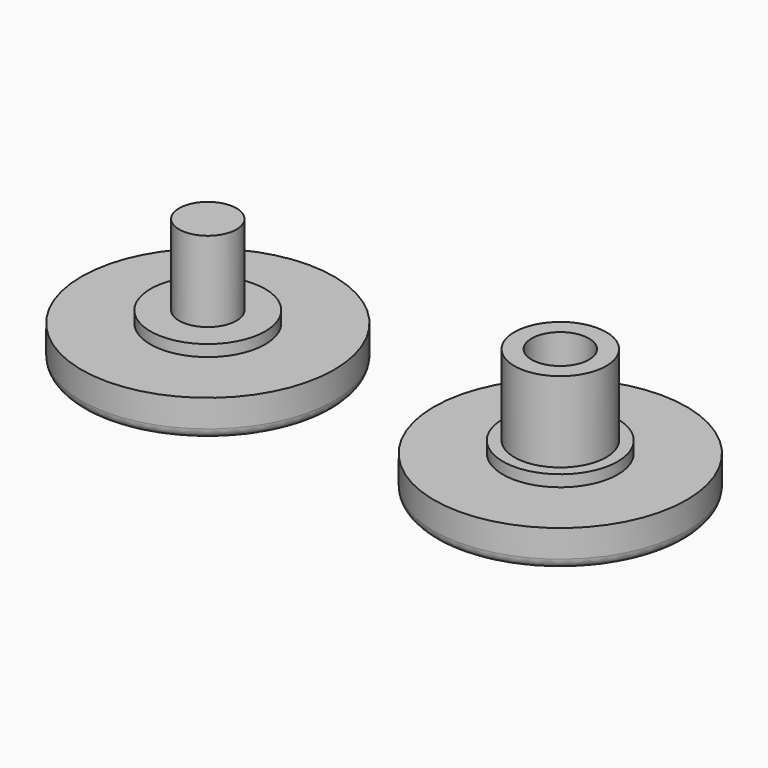
from build123d import *

# Parameters (mm, degrees)
F0_R      = 11
F1_DEPTH  = 3.5
F2_R      = 5
F3_DEPTH  = 1
F4_R      = 4
F5_DEPTH  = 7
F6_R      = 1.3518679975
F7_DEPTH  = 32.3
F11_R     = 0.9092071391
F13_R     = 2.5
F14_DEPTH = 7
F15_R     = 4
F15_R_2   = 2.5
F16_DEPTH = 7


# Not quite as in the source:
# - a fillet or chamfer that OpenCascade refuses, or shapes differently, is made with other operations: its cross-section is extruded or revolved along the edge and cut away or added
# - a feature names something its author has since deleted; it is built from what else it names


with BuildPart() as f1:
    # F0 (on Top) → F1 (new body)
    with BuildSketch(Plane.XY):
        with Locations((59.4149753451, 64.0600547194)):
            Circle(F0_R)
    extrude(amount=F1_DEPTH)

    # F2 (on face) → F3 (join)
    with BuildSketch(Plane.XY.offset(3.5)):
        with Locations((59.4149753451, 64.0600547194)):
            Circle(F2_R)
    extrude(amount=F3_DEPTH)

    # F4 (on face) → F5 (join)
    with BuildSketch(Plane.XY.offset(4.5)):
        with Locations((59.4149753451, 64.0600547194)):
            Circle(F4_R)
    extrude(amount=F5_DEPTH)

    # F6 (on face) → F7 (join)
    with BuildSketch(Plane(origin=(0, 0, 0), x_dir=(1, 0, 0), z_dir=(0, 0, -1))):
        with Locations((59.4149753451, -64.0600547194)):
            Circle(F6_R)
    extrude(amount=F7_DEPTH)

    # F8 (on face) → F9 (revolve, cut)
    with BuildSketch(Plane(origin=(0, 0, -32.3), x_dir=(1, 0, 0), z_dir=(0, 0, -1))):
        with BuildLine():
            Line((60.7668433426, -64.0600547194), (93.4149753451, -64.0600547194))
            ThreePointArc((93.4149753451, -64.0600547194), (59.4149753451, -30.0600547194), (25.4149753451, -64.0600547194))
            Line((25.4149753451, -64.0600547194), (58.0631073476, -64.0600547194))
            ThreePointArc((58.0631073476, -64.0600547194), (59.4149753451, -62.7081867219), (60.7668433426, -64.0600547194))
        make_face()
        with BuildLine():
            Line((59.4149753451, -64.0600547194), (60.7668433426, -64.0600547194))
            ThreePointArc((60.7668433426, -64.0600547194), (59.4149753451, -62.7081867219), (58.0631073476, -64.0600547194))
            Line((58.0631073476, -64.0600547194), (59.4149753451, -64.0600547194))
        make_face()
    revolve(axis=Axis((76.4149753451, 64.0600547194, -32.3), (1, 0, 0)), mode=Mode.SUBTRACT)

    # F10: fillet of radius 5 on 1 edges, made by hand

    # F10_s1 → F10_t2 (revolve, cut)
    with BuildSketch(Plane.YZ.offset(59.4149753451)):
        with BuildLine():
            ThreePointArc((52.67102491, 0), (53.4091792265, 0.0547873448), (54.1311569369, 0.2179487179))
            ThreePointArc((54.1311569369, 0.2179487179), (53.7867795374, 0.1107978463), (53.4435581222, 0))
            Line((53.4435581222, 0), (52.67102491, 0))
        make_face()
    revolve(axis=Axis((59.4149753451, 64.0600547194, 0), (0, 0, 1)), mode=Mode.SUBTRACT)

    # F11
    f11_edges = [f1.edges().sort_by_distance(p)[0] for p in [
        (51.636801, 71.838229, 0.015157),
        (67.19315, 56.28188, 0.015157),
    ]]
    fillet(f11_edges, radius=F11_R)


with BuildPart() as f12_1:
    # F12: copy of F1
    add(f1.part.moved(Location((-30.7, 0, 0))))

    # F15 (on face) → F16 (cut)
    with BuildSketch(Plane.XY.offset(11.5)):
        with Locations((28.7149753451, 64.0600547194)):
            Circle(F15_R)
        with Locations((28.7149753451, 64.0600547194)):
            Circle(F15_R_2, mode=Mode.SUBTRACT)
    extrude(amount=-F16_DEPTH, mode=Mode.SUBTRACT)


with BuildPart() as f1_1:
    add(f1.part)

    # F13 (on face) → F14 (cut)
    with BuildSketch(Plane.XY.offset(11.5)):
        with Locations((59.4149753451, 64.0600547194)):
            Circle(F13_R)
    extrude(amount=-F14_DEPTH, mode=Mode.SUBTRACT)


solid = Compound([f12_1.part, f1_1.part])
